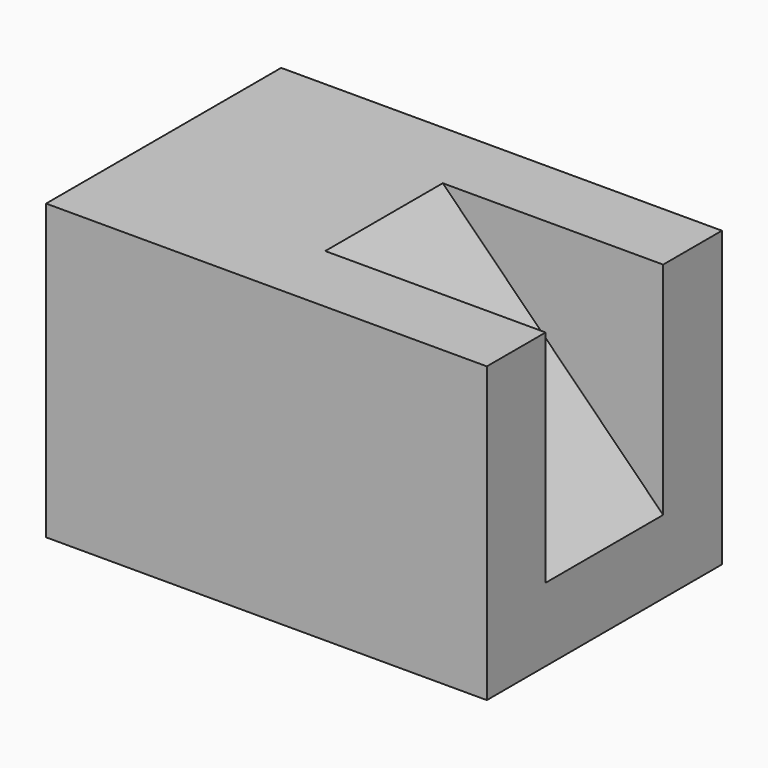
from build123d import *

# Parameters (mm, degrees)
F0_W      = 38.1
F0_H      = 25.4
F1_DEPTH  = 25.4
F3_DEPTH  = 25.401
F4_W      = 20.8833201349
F4_H      = 7.9113657147
F4_H_2    = 6.35
F5_DEPTH  = 25.4
F7_DEPTH  = 25.4
F10_W     = 2.4862326682
F10_H     = 25.8971806616
F11_DEPTH = 26.9623657147


# Not quite as in the source:
# - a feature of the source that left no trace in its solid (it failed there, or was rolled back) is left out


with BuildPart() as f1:
    # F0 (on Front) → F1 (new body)
    with BuildSketch(Plane.XZ):
        with Locations((19.05, -12.7)):
            Rectangle(F0_W, F0_H)
    extrude(amount=F1_DEPTH)

    # F2 (on Front) → F3 (cut, through all)
    with BuildSketch(Plane.XZ):
        Polygon((38.1, 0), (19.05, 0), (38.1, -19.05), align=None)
    extrude(amount=F3_DEPTH, mode=Mode.SUBTRACT)

    # F4 (on Top) → F5 (join)
    with BuildSketch(Plane.XY):
        with Locations((29.4916600674, -23.0056828573)):
            Rectangle(F4_W, F4_H)
        with Locations((29.4916600674, -3.175)):
            Rectangle(F4_W, F4_H_2)
    extrude(amount=-F5_DEPTH)

    # F6 (on Top) → F7 (cut)
    with BuildSketch(Plane.XY):
        Polygon((38.1, -25.4), (18.3193590492, -25.4), (18.3193590492, -27.6306644082), (39.8231558502, -27.6306644082), (39.8231558502, 0), (38.1, 0), align=None)
    extrude(amount=-F7_DEPTH, mode=Mode.SUBTRACT)

    # F10 (on Front) → F11 (cut, through all)
    with BuildSketch(Plane.XZ):
        with Locations((40.0636065751, -12.9485903308)):
            Rectangle(F10_W, F10_H)
    extrude(amount=F11_DEPTH, mode=Mode.SUBTRACT)


solid = f1.part
